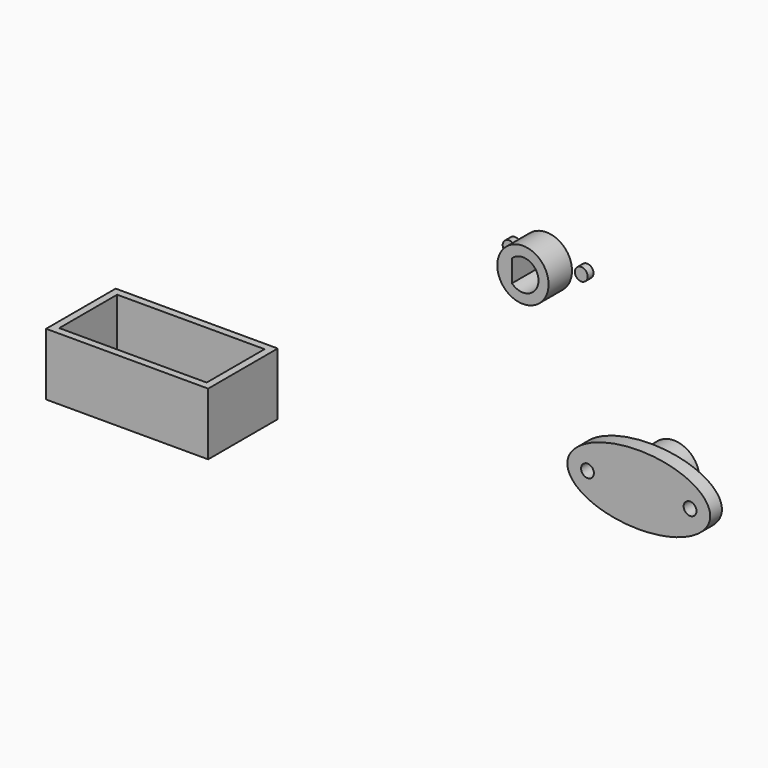
from build123d import *

# Parameters (mm, degrees)
F0_R      = 7
F1_DEPTH  = 8
F3_DEPTH  = 4
F4_R      = 1.75
F5_DEPTH  = 4
F7_DEPTH  = 8
F8_W      = 44.25
F8_H      = 23.75
F8_W_2    = 40.25
F8_H_2    = 19.75
F9_DEPTH  = 17
F10_R     = 7
F11_DEPTH = 8
F12_R     = 1.75
F13_DEPTH = 2


with BuildPart() as f1:
    # F0 (on Front) → F1 (new body)
    with BuildSketch(Plane.XZ):
        Circle(F0_R)
    extrude(amount=F1_DEPTH)

    # F2 (on face) → F3 (join)
    with BuildSketch(Plane.XZ.offset(8)):
        with BuildLine():
            add(Edge.make_bspline(
                [(-19.5, 0), (-19.5, -16.4544826719), (9.75, -8.227241336), (39, 0), (9.75, 8.227241336), (-19.5, 16.4544826719), (-19.5, 0)],
                knots=[0, 0, 0, 2.0943951024, 2.0943951024, 4.1887902048, 4.1887902048, 6.2831853072, 6.2831853072, 6.2831853072], degree=2, weights=[1, 0.5, 1, 0.5, 1, 0.5, 1]))
        make_face()
    extrude(amount=F3_DEPTH)

    # F4 (on face) → F5 (cut)
    with BuildSketch(Plane.XZ.offset(12)):
        with Locations((-14, 0)):
            Circle(F4_R)
        with Locations((14, 0)):
            Circle(F4_R)
    extrude(amount=-F5_DEPTH, mode=Mode.SUBTRACT)

    # F6 (on face) → F7 (cut)
    with BuildSketch(Plane(origin=(0, 0, 0), x_dir=(-1, 0, 0), z_dir=(0, 1, 0))):
        with BuildLine():
            ThreePointArc((-3, -3.0103986447), (1.6298006013, -3.925079617), (4.25, 0))
            ThreePointArc((4.25, 0), (1.6298006013, 3.925079617), (-3, 3.0103986447))
            Line((-3, 3.0103986447), (-3, 0))
            Line((-3, 0), (-3, -3.0103986447))
        make_face()
    extrude(amount=-F7_DEPTH, mode=Mode.SUBTRACT)


with BuildPart() as f9:
    # F8 (on Top) → F9 (new body)
    with BuildSketch(Plane.XY):
        with Locations((-102.5861466527, -46.512093246)):
            Rectangle(F8_W, F8_H)
        with Locations((-102.5861466527, -46.512093246)):
            Rectangle(F8_W_2, F8_H_2, mode=Mode.SUBTRACT)
    extrude(amount=F9_DEPTH)


with BuildPart() as f11:
    # F10 (on Front) → F11 (new body)
    with BuildSketch(Plane.XZ):
        with Locations((-34.8314889967, 38.7026694899)):
            Circle(F10_R)
        with BuildLine():
            ThreePointArc((-37.8314889967, 41.7130681346), (-33.2016883954, 42.6277491069), (-30.5814889967, 38.7026694899))
            ThreePointArc((-30.5814889967, 38.7026694899), (-33.2016883954, 34.7775898728), (-37.8314889967, 35.6922708452))
            ThreePointArc((-37.8314889967, 35.6922708452), (-39.0814889967, 38.7026694899), (-37.8314889967, 41.7130681346))
        make_face(mode=Mode.SUBTRACT)
        with BuildLine():
            Line((-37.8314889967, 38.7026694899), (-37.8314889967, 41.7130681346))
            ThreePointArc((-37.8314889967, 41.7130681346), (-39.0814889967, 38.7026694899), (-37.8314889967, 35.6922708452))
            Line((-37.8314889967, 35.6922708452), (-37.8314889967, 38.7026694899))
        make_face()
    extrude(amount=F11_DEPTH)


with BuildPart() as f13:
    # F12 (on face) → F13 (new body)
    with BuildSketch(Plane(origin=(0, 0, 0), x_dir=(-1, 0, 0), z_dir=(0, 1, 0))):
        with Locations((25.309631601, 38.7026694899)):
            Circle(F12_R)
    extrude(amount=F13_DEPTH)


with BuildPart() as f13b:
    # F12 (on face) → F13, piece 2 (new body)
    with BuildSketch(Plane(origin=(0, 0, 0), x_dir=(-1, 0, 0), z_dir=(0, 1, 0))):
        with Locations((45.0074523687, 38.7026694899)):
            Circle(F12_R)
    extrude(amount=F13_DEPTH)


solid = Compound([f1.part, f9.part, f11.part, f13.part, f13b.part])
